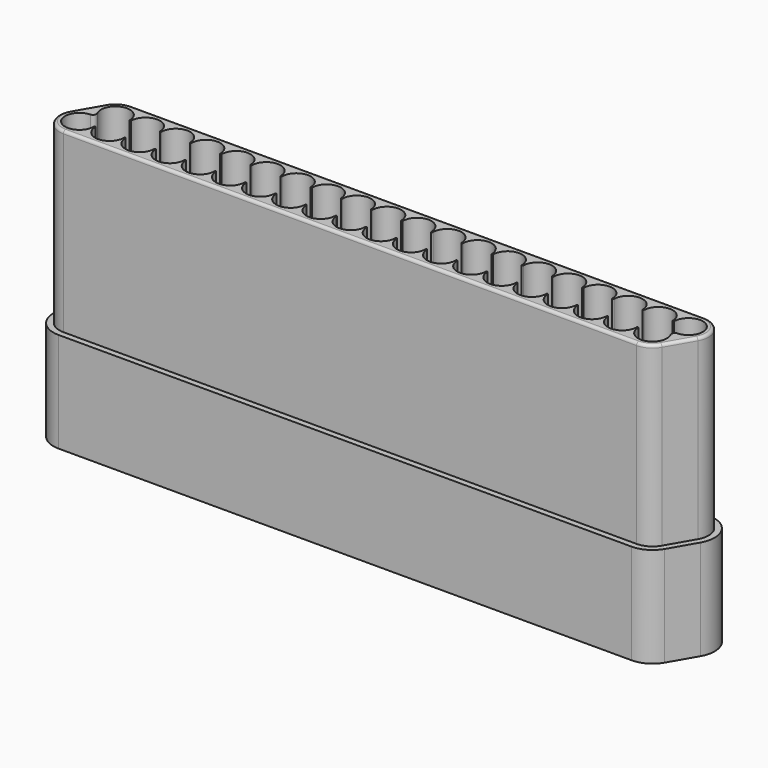
from build123d import *

# Parameters (mm, degrees)
F1_DEPTH = 75
F2_DEPTH = 25
F3_DEPTH = 3.2
F4_R     = 0.8


# Not quite as in the source:
# - a feature names something its author has since deleted; it is built from what else it names


with BuildPart() as f1:
    # F0 (on Top) → F1 (new body)
    with BuildSketch(Plane.XY):
        with BuildLine():
            Line((-0.6430435314, 10.1862159322), (-4.8930435314, 2.825))
            ThreePointArc((-4.8930435314, 2.825), (-4.8930435314, -2.825), (0, -5.65))
            Line((0, -5.65), (161.5, -5.65))
            ThreePointArc((161.5, -5.65), (164.325, -4.8930435314), (166.3930435314, -2.825))
            Line((166.3930435314, -2.825), (170.6430435314, 4.5362159322))
            ThreePointArc((170.6430435314, 4.5362159322), (170.6430435314, 10.1862159322), (165.75, 13.0112159322))
            Line((165.75, 13.0112159322), (4.25, 13.0112159322))
            ThreePointArc((4.25, 13.0112159322), (1.425, 12.2542594635), (-0.6430435314, 10.1862159322))
        make_face()
        with BuildLine():
            ThreePointArc((4.45, 0), (4.25, -0.2), (4.05, 0))
            ThreePointArc((4.05, 0), (-2.7957165477, -2.9302677326), (-0.1902315974, 4.0455298713))
            ThreePointArc((-0.1902315974, 4.0455298713), (0.6288230416, 4.5444261358), (0.651352561, 5.5031963925))
            ThreePointArc((0.651352561, 5.5031963925), (3.2939723142, 11.2967605024), (8.3, 7.3612159322))
            ThreePointArc((8.3, 7.3612159322), (8.5, 7.5612159322), (8.7, 7.3612159322))
            ThreePointArc((8.7, 7.3612159322), (12.75, 11.4112159322), (16.8, 7.3612159322))
            ThreePointArc((16.8, 7.3612159322), (17, 7.5612159322), (17.2, 7.3612159322))
            ThreePointArc((17.2, 7.3612159322), (21.25, 11.4112159322), (25.3, 7.3612159322))
            ThreePointArc((25.3, 7.3612159322), (25.5, 7.5612159322), (25.7, 7.3612159322))
            ThreePointArc((25.7, 7.3612159322), (29.75, 11.4112159322), (33.8, 7.3612159322))
            ThreePointArc((33.8, 7.3612159322), (34, 7.5612159322), (34.2, 7.3612159322))
            ThreePointArc((34.2, 7.3612159322), (38.25, 11.4112159322), (42.3, 7.3612159322))
            ThreePointArc((42.3, 7.3612159322), (42.5, 7.5612159322), (42.7, 7.3612159322))
            ThreePointArc((42.7, 7.3612159322), (46.75, 11.4112159322), (50.8, 7.3612159322))
            ThreePointArc((50.8, 7.3612159322), (51, 7.5612159322), (51.2, 7.3612159322))
            ThreePointArc((51.2, 7.3612159322), (55.25, 11.4112159322), (59.3, 7.3612159322))
            ThreePointArc((59.3, 7.3612159322), (59.5, 7.5612159322), (59.7, 7.3612159322))
            ThreePointArc((59.7, 7.3612159322), (63.75, 11.4112159322), (67.8, 7.3612159322))
            ThreePointArc((67.8, 7.3612159322), (68, 7.5612159322), (68.2, 7.3612159322))
            ThreePointArc((68.2, 7.3612159322), (72.25, 11.4112159322), (76.3, 7.3612159322))
            ThreePointArc((76.3, 7.3612159322), (76.5, 7.5612159322), (76.7, 7.3612159322))
            ThreePointArc((76.7, 7.3612159322), (80.75, 11.4112159322), (84.8, 7.3612159322))
            ThreePointArc((84.8, 7.3612159322), (85, 7.5612159322), (85.2, 7.3612159322))
            ThreePointArc((85.2, 7.3612159322), (89.25, 11.4112159322), (93.3, 7.3612159322))
            ThreePointArc((93.3, 7.3612159322), (93.5, 7.5612159322), (93.7, 7.3612159322))
            ThreePointArc((93.7, 7.3612159322), (97.75, 11.4112159322), (101.8, 7.3612159322))
            ThreePointArc((101.8, 7.3612159322), (102, 7.5612159322), (102.2, 7.3612159322))
            ThreePointArc((102.2, 7.3612159322), (106.25, 11.4112159322), (110.3, 7.3612159322))
            ThreePointArc((110.3, 7.3612159322), (110.5, 7.5612159322), (110.7, 7.3612159322))
            ThreePointArc((110.7, 7.3612159322), (114.75, 11.4112159322), (118.8, 7.3612159322))
            ThreePointArc((118.8, 7.3612159322), (119, 7.5612159322), (119.2, 7.3612159322))
            ThreePointArc((119.2, 7.3612159322), (123.25, 11.4112159322), (127.3, 7.3612159322))
            ThreePointArc((127.3, 7.3612159322), (127.5, 7.5612159322), (127.7, 7.3612159322))
            ThreePointArc((127.7, 7.3612159322), (131.75, 11.4112159322), (135.8, 7.3612159322))
            ThreePointArc((135.8, 7.3612159322), (136, 7.5612159322), (136.2, 7.3612159322))
            ThreePointArc((136.2, 7.3612159322), (140.25, 11.4112159322), (144.3, 7.3612159322))
            ThreePointArc((144.3, 7.3612159322), (144.5, 7.5612159322), (144.7, 7.3612159322))
            ThreePointArc((144.7, 7.3612159322), (148.75, 11.4112159322), (152.8, 7.3612159322))
            ThreePointArc((152.8, 7.3612159322), (153, 7.5612159322), (153.2, 7.3612159322))
            ThreePointArc((153.2, 7.3612159322), (157.25, 11.4112159322), (161.3, 7.3612159322))
            ThreePointArc((161.3, 7.3612159322), (161.5, 7.5612159322), (161.7, 7.3612159322))
            ThreePointArc((161.7, 7.3612159322), (165.75, 11.4112159322), (169.8, 7.3612159322))
            ThreePointArc((169.8, 7.3612159322), (168.6802677326, 4.5654993844), (165.9402315974, 3.3156860609))
            ThreePointArc((165.9402315974, 3.3156860609), (165.1211769584, 2.8167897964), (165.098647439, 1.8580195397))
            ThreePointArc((165.098647439, 1.8580195397), (165.4355445702, 0.9560276858), (165.55, 0))
            ThreePointArc((165.55, 0), (161.5, -4.05), (157.45, 0))
            ThreePointArc((157.45, 0), (157.25, -0.2), (157.05, 0))
            ThreePointArc((157.05, 0), (153, -4.05), (148.95, 0))
            ThreePointArc((148.95, 0), (148.75, -0.2), (148.55, 0))
            ThreePointArc((148.55, 0), (144.5, -4.05), (140.45, 0))
            ThreePointArc((140.45, 0), (140.25, -0.2), (140.05, 0))
            ThreePointArc((140.05, 0), (136, -4.05), (131.95, 0))
            ThreePointArc((131.95, 0), (131.75, -0.2), (131.55, 0))
            ThreePointArc((131.55, 0), (127.5, -4.05), (123.45, 0))
            ThreePointArc((123.45, 0), (123.25, -0.2), (123.05, 0))
            ThreePointArc((123.05, 0), (119, -4.05), (114.95, 0))
            ThreePointArc((114.95, 0), (114.75, -0.2), (114.55, 0))
            ThreePointArc((114.55, 0), (110.5, -4.05), (106.45, 0))
            ThreePointArc((106.45, 0), (106.25, -0.2), (106.05, 0))
            ThreePointArc((106.05, 0), (102, -4.05), (97.95, 0))
            ThreePointArc((97.95, 0), (97.75, -0.2), (97.55, 0))
            ThreePointArc((97.55, 0), (93.5, -4.05), (89.45, 0))
            ThreePointArc((89.45, 0), (89.25, -0.2), (89.05, 0))
            ThreePointArc((89.05, 0), (85, -4.05), (80.95, 0))
            ThreePointArc((80.95, 0), (80.75, -0.2), (80.55, 0))
            ThreePointArc((80.55, 0), (76.5, -4.05), (72.45, 0))
            ThreePointArc((72.45, 0), (72.25, -0.2), (72.05, 0))
            ThreePointArc((72.05, 0), (68, -4.05), (63.95, 0))
            ThreePointArc((63.95, 0), (63.75, -0.2), (63.55, 0))
            ThreePointArc((63.55, 0), (59.5, -4.05), (55.45, 0))
            ThreePointArc((55.45, 0), (55.25, -0.2), (55.05, 0))
            ThreePointArc((55.05, 0), (51, -4.05), (46.95, 0))
            ThreePointArc((46.95, 0), (46.75, -0.2), (46.55, 0))
            ThreePointArc((46.55, 0), (42.5, -4.05), (38.45, 0))
            ThreePointArc((38.45, 0), (38.25, -0.2), (38.05, 0))
            ThreePointArc((38.05, 0), (34, -4.05), (29.95, 0))
            ThreePointArc((29.95, 0), (29.75, -0.2), (29.55, 0))
            ThreePointArc((29.55, 0), (25.5, -4.05), (21.45, 0))
            ThreePointArc((21.45, 0), (21.25, -0.2), (21.05, 0))
            ThreePointArc((21.05, 0), (17, -4.05), (12.95, 0))
            ThreePointArc((12.95, 0), (12.75, -0.2), (12.55, 0))
            ThreePointArc((12.55, 0), (8.5, -4.05), (4.45, 0))
        make_face(mode=Mode.SUBTRACT)
        with BuildLine():
            ThreePointArc((4.45, 0), (4.25, 0.2), (4.05, 0))
            ThreePointArc((4.05, 0), (4.25, -0.2), (4.45, 0))
        make_face()
        with BuildLine():
            ThreePointArc((8.7, 7.3612159322), (8.5, 7.5612159322), (8.3, 7.3612159322))
            ThreePointArc((8.3, 7.3612159322), (8.5, 7.1612159322), (8.7, 7.3612159322))
        make_face()
        with BuildLine():
            ThreePointArc((12.95, 0), (12.75, 0.2), (12.55, 0))
            ThreePointArc((12.55, 0), (12.75, -0.2), (12.95, 0))
        make_face()
        with BuildLine():
            ThreePointArc((17.2, 7.3612159322), (17, 7.5612159322), (16.8, 7.3612159322))
            ThreePointArc((16.8, 7.3612159322), (17, 7.1612159322), (17.2, 7.3612159322))
        make_face()
        with BuildLine():
            ThreePointArc((21.45, 0), (21.25, 0.2), (21.05, 0))
            ThreePointArc((21.05, 0), (21.25, -0.2), (21.45, 0))
        make_face()
        with BuildLine():
            ThreePointArc((25.7, 7.3612159322), (25.5, 7.5612159322), (25.3, 7.3612159322))
            ThreePointArc((25.3, 7.3612159322), (25.5, 7.1612159322), (25.7, 7.3612159322))
        make_face()
        with BuildLine():
            ThreePointArc((29.95, 0), (29.75, 0.2), (29.55, 0))
            ThreePointArc((29.55, 0), (29.75, -0.2), (29.95, 0))
        make_face()
        with BuildLine():
            ThreePointArc((34.2, 7.3612159322), (34, 7.5612159322), (33.8, 7.3612159322))
            ThreePointArc((33.8, 7.3612159322), (34, 7.1612159322), (34.2, 7.3612159322))
        make_face()
        with BuildLine():
            ThreePointArc((38.45, 0), (38.25, 0.2), (38.05, 0))
            ThreePointArc((38.05, 0), (38.25, -0.2), (38.45, 0))
        make_face()
        with BuildLine():
            ThreePointArc((42.7, 7.3612159322), (42.5, 7.5612159322), (42.3, 7.3612159322))
            ThreePointArc((42.3, 7.3612159322), (42.5, 7.1612159322), (42.7, 7.3612159322))
        make_face()
        with BuildLine():
            ThreePointArc((46.95, 0), (46.75, 0.2), (46.55, 0))
            ThreePointArc((46.55, 0), (46.75, -0.2), (46.95, 0))
        make_face()
        with BuildLine():
            ThreePointArc((51.2, 7.3612159322), (51, 7.5612159322), (50.8, 7.3612159322))
            ThreePointArc((50.8, 7.3612159322), (51, 7.1612159322), (51.2, 7.3612159322))
        make_face()
        with BuildLine():
            ThreePointArc((55.45, 0), (55.25, 0.2), (55.05, 0))
            ThreePointArc((55.05, 0), (55.25, -0.2), (55.45, 0))
        make_face()
        with BuildLine():
            ThreePointArc((59.7, 7.3612159322), (59.5, 7.5612159322), (59.3, 7.3612159322))
            ThreePointArc((59.3, 7.3612159322), (59.5, 7.1612159322), (59.7, 7.3612159322))
        make_face()
        with BuildLine():
            ThreePointArc((63.95, 0), (63.75, 0.2), (63.55, 0))
            ThreePointArc((63.55, 0), (63.75, -0.2), (63.95, 0))
        make_face()
        with BuildLine():
            ThreePointArc((68.2, 7.3612159322), (68, 7.5612159322), (67.8, 7.3612159322))
            ThreePointArc((67.8, 7.3612159322), (68, 7.1612159322), (68.2, 7.3612159322))
        make_face()
        with BuildLine():
            ThreePointArc((72.45, 0), (72.25, 0.2), (72.05, 0))
            ThreePointArc((72.05, 0), (72.25, -0.2), (72.45, 0))
        make_face()
        with BuildLine():
            ThreePointArc((76.7, 7.3612159322), (76.5, 7.5612159322), (76.3, 7.3612159322))
            ThreePointArc((76.3, 7.3612159322), (76.5, 7.1612159322), (76.7, 7.3612159322))
        make_face()
        with BuildLine():
            ThreePointArc((80.95, 0), (80.75, 0.2), (80.55, 0))
            ThreePointArc((80.55, 0), (80.75, -0.2), (80.95, 0))
        make_face()
        with BuildLine():
            ThreePointArc((85.2, 7.3612159322), (85, 7.5612159322), (84.8, 7.3612159322))
            ThreePointArc((84.8, 7.3612159322), (85, 7.1612159322), (85.2, 7.3612159322))
        make_face()
        with BuildLine():
            ThreePointArc((89.45, 0), (89.25, 0.2), (89.05, 0))
            ThreePointArc((89.05, 0), (89.25, -0.2), (89.45, 0))
        make_face()
        with BuildLine():
            ThreePointArc((93.7, 7.3612159322), (93.5, 7.5612159322), (93.3, 7.3612159322))
            ThreePointArc((93.3, 7.3612159322), (93.5, 7.1612159322), (93.7, 7.3612159322))
        make_face()
        with BuildLine():
            ThreePointArc((97.95, 0), (97.75, 0.2), (97.55, 0))
            ThreePointArc((97.55, 0), (97.75, -0.2), (97.95, 0))
        make_face()
        with BuildLine():
            ThreePointArc((102.2, 7.3612159322), (102, 7.5612159322), (101.8, 7.3612159322))
            ThreePointArc((101.8, 7.3612159322), (102, 7.1612159322), (102.2, 7.3612159322))
        make_face()
        with BuildLine():
            ThreePointArc((106.45, 0), (106.25, 0.2), (106.05, 0))
            ThreePointArc((106.05, 0), (106.25, -0.2), (106.45, 0))
        make_face()
        with BuildLine():
            ThreePointArc((110.7, 7.3612159322), (110.5, 7.5612159322), (110.3, 7.3612159322))
            ThreePointArc((110.3, 7.3612159322), (110.5, 7.1612159322), (110.7, 7.3612159322))
        make_face()
        with BuildLine():
            ThreePointArc((114.95, 0), (114.75, 0.2), (114.55, 0))
            ThreePointArc((114.55, 0), (114.75, -0.2), (114.95, 0))
        make_face()
        with BuildLine():
            ThreePointArc((119.2, 7.3612159322), (119, 7.5612159322), (118.8, 7.3612159322))
            ThreePointArc((118.8, 7.3612159322), (119, 7.1612159322), (119.2, 7.3612159322))
        make_face()
        with BuildLine():
            ThreePointArc((123.45, 0), (123.25, 0.2), (123.05, 0))
            ThreePointArc((123.05, 0), (123.25, -0.2), (123.45, 0))
        make_face()
        with BuildLine():
            ThreePointArc((127.7, 7.3612159322), (127.5, 7.5612159322), (127.3, 7.3612159322))
            ThreePointArc((127.3, 7.3612159322), (127.5, 7.1612159322), (127.7, 7.3612159322))
        make_face()
        with BuildLine():
            ThreePointArc((131.95, 0), (131.75, 0.2), (131.55, 0))
            ThreePointArc((131.55, 0), (131.75, -0.2), (131.95, 0))
        make_face()
        with BuildLine():
            ThreePointArc((136.2, 7.3612159322), (136, 7.5612159322), (135.8, 7.3612159322))
            ThreePointArc((135.8, 7.3612159322), (136, 7.1612159322), (136.2, 7.3612159322))
        make_face()
        with BuildLine():
            ThreePointArc((140.45, 0), (140.25, 0.2), (140.05, 0))
            ThreePointArc((140.05, 0), (140.25, -0.2), (140.45, 0))
        make_face()
        with BuildLine():
            ThreePointArc((144.7, 7.3612159322), (144.5, 7.5612159322), (144.3, 7.3612159322))
            ThreePointArc((144.3, 7.3612159322), (144.5, 7.1612159322), (144.7, 7.3612159322))
        make_face()
        with BuildLine():
            ThreePointArc((148.95, 0), (148.75, 0.2), (148.55, 0))
            ThreePointArc((148.55, 0), (148.75, -0.2), (148.95, 0))
        make_face()
        with BuildLine():
            ThreePointArc((153.2, 7.3612159322), (153, 7.5612159322), (152.8, 7.3612159322))
            ThreePointArc((152.8, 7.3612159322), (153, 7.1612159322), (153.2, 7.3612159322))
        make_face()
        with BuildLine():
            ThreePointArc((157.45, 0), (157.25, 0.2), (157.05, 0))
            ThreePointArc((157.05, 0), (157.25, -0.2), (157.45, 0))
        make_face()
        with BuildLine():
            ThreePointArc((161.7, 7.3612159322), (161.5, 7.5612159322), (161.3, 7.3612159322))
            ThreePointArc((161.3, 7.3612159322), (161.5, 7.1612159322), (161.7, 7.3612159322))
        make_face()
    extrude(amount=F1_DEPTH)

    # F0 (on Top) → F2 (join)
    with BuildSketch(Plane.XY):
        with BuildLine():
            Line((-2.1152867178, 11.0362159322), (-6.3652867178, 3.675))
            ThreePointArc((-6.3652867178, 3.675), (-6.3652867178, -3.675), (0, -7.35))
            Line((0, -7.35), (161.5, -7.35))
            ThreePointArc((161.5, -7.35), (165.175, -6.3652867178), (167.8652867178, -3.675))
            Line((167.8652867178, -3.675), (172.1152867178, 3.6862159322))
            ThreePointArc((172.1152867178, 3.6862159322), (172.1152867178, 11.0362159322), (165.75, 14.7112159322))
            Line((165.75, 14.7112159322), (4.25, 14.7112159322))
            ThreePointArc((4.25, 14.7112159322), (0.575, 13.72650265), (-2.1152867178, 11.0362159322))
        make_face()
        with BuildLine():
            ThreePointArc((0, -5.65), (-4.8930435314, -2.825), (-4.8930435314, 2.825))
            Line((-4.8930435314, 2.825), (-0.6430435314, 10.1862159322))
            ThreePointArc((-0.6430435314, 10.1862159322), (1.425, 12.2542594635), (4.25, 13.0112159322))
            Line((4.25, 13.0112159322), (165.75, 13.0112159322))
            ThreePointArc((165.75, 13.0112159322), (170.6430435314, 10.1862159322), (170.6430435314, 4.5362159322))
            Line((170.6430435314, 4.5362159322), (166.3930435314, -2.825))
            ThreePointArc((166.3930435314, -2.825), (164.325, -4.8930435314), (161.5, -5.65))
            Line((161.5, -5.65), (0, -5.65))
        make_face(mode=Mode.SUBTRACT)
    extrude(amount=F2_DEPTH)

    # F0 (on Top) → F3 (join)
    with BuildSketch(Plane.XY):
        with BuildLine():
            Line((-2.1152867178, 11.0362159322), (-6.3652867178, 3.675))
            ThreePointArc((-6.3652867178, 3.675), (-6.3652867178, -3.675), (0, -7.35))
            Line((0, -7.35), (161.5, -7.35))
            ThreePointArc((161.5, -7.35), (165.175, -6.3652867178), (167.8652867178, -3.675))
            Line((167.8652867178, -3.675), (172.1152867178, 3.6862159322))
            ThreePointArc((172.1152867178, 3.6862159322), (172.1152867178, 11.0362159322), (165.75, 14.7112159322))
            Line((165.75, 14.7112159322), (4.25, 14.7112159322))
            ThreePointArc((4.25, 14.7112159322), (0.575, 13.72650265), (-2.1152867178, 11.0362159322))
        make_face()
        with BuildLine():
            ThreePointArc((0, -5.65), (-4.8930435314, -2.825), (-4.8930435314, 2.825))
            Line((-4.8930435314, 2.825), (-0.6430435314, 10.1862159322))
            ThreePointArc((-0.6430435314, 10.1862159322), (1.425, 12.2542594635), (4.25, 13.0112159322))
            Line((4.25, 13.0112159322), (165.75, 13.0112159322))
            ThreePointArc((165.75, 13.0112159322), (170.6430435314, 10.1862159322), (170.6430435314, 4.5362159322))
            Line((170.6430435314, 4.5362159322), (166.3930435314, -2.825))
            ThreePointArc((166.3930435314, -2.825), (164.325, -4.8930435314), (161.5, -5.65))
            Line((161.5, -5.65), (0, -5.65))
        make_face(mode=Mode.SUBTRACT)
        with BuildLine():
            Line((-0.6430435314, 10.1862159322), (-4.8930435314, 2.825))
            ThreePointArc((-4.8930435314, 2.825), (-4.8930435314, -2.825), (0, -5.65))
            Line((0, -5.65), (161.5, -5.65))
            ThreePointArc((161.5, -5.65), (164.325, -4.8930435314), (166.3930435314, -2.825))
            Line((166.3930435314, -2.825), (170.6430435314, 4.5362159322))
            ThreePointArc((170.6430435314, 4.5362159322), (170.6430435314, 10.1862159322), (165.75, 13.0112159322))
            Line((165.75, 13.0112159322), (4.25, 13.0112159322))
            ThreePointArc((4.25, 13.0112159322), (1.425, 12.2542594635), (-0.6430435314, 10.1862159322))
        make_face()
        with BuildLine():
            ThreePointArc((4.45, 0), (4.25, -0.2), (4.05, 0))
            ThreePointArc((4.05, 0), (-2.7957165477, -2.9302677326), (-0.1902315974, 4.0455298713))
            ThreePointArc((-0.1902315974, 4.0455298713), (0.6288230416, 4.5444261358), (0.651352561, 5.5031963925))
            ThreePointArc((0.651352561, 5.5031963925), (3.2939723142, 11.2967605024), (8.3, 7.3612159322))
            ThreePointArc((8.3, 7.3612159322), (8.5, 7.5612159322), (8.7, 7.3612159322))
            ThreePointArc((8.7, 7.3612159322), (12.75, 11.4112159322), (16.8, 7.3612159322))
            ThreePointArc((16.8, 7.3612159322), (17, 7.5612159322), (17.2, 7.3612159322))
            ThreePointArc((17.2, 7.3612159322), (21.25, 11.4112159322), (25.3, 7.3612159322))
            ThreePointArc((25.3, 7.3612159322), (25.5, 7.5612159322), (25.7, 7.3612159322))
            ThreePointArc((25.7, 7.3612159322), (29.75, 11.4112159322), (33.8, 7.3612159322))
            ThreePointArc((33.8, 7.3612159322), (34, 7.5612159322), (34.2, 7.3612159322))
            ThreePointArc((34.2, 7.3612159322), (38.25, 11.4112159322), (42.3, 7.3612159322))
            ThreePointArc((42.3, 7.3612159322), (42.5, 7.5612159322), (42.7, 7.3612159322))
            ThreePointArc((42.7, 7.3612159322), (46.75, 11.4112159322), (50.8, 7.3612159322))
            ThreePointArc((50.8, 7.3612159322), (51, 7.5612159322), (51.2, 7.3612159322))
            ThreePointArc((51.2, 7.3612159322), (55.25, 11.4112159322), (59.3, 7.3612159322))
            ThreePointArc((59.3, 7.3612159322), (59.5, 7.5612159322), (59.7, 7.3612159322))
            ThreePointArc((59.7, 7.3612159322), (63.75, 11.4112159322), (67.8, 7.3612159322))
            ThreePointArc((67.8, 7.3612159322), (68, 7.5612159322), (68.2, 7.3612159322))
            ThreePointArc((68.2, 7.3612159322), (72.25, 11.4112159322), (76.3, 7.3612159322))
            ThreePointArc((76.3, 7.3612159322), (76.5, 7.5612159322), (76.7, 7.3612159322))
            ThreePointArc((76.7, 7.3612159322), (80.75, 11.4112159322), (84.8, 7.3612159322))
            ThreePointArc((84.8, 7.3612159322), (85, 7.5612159322), (85.2, 7.3612159322))
            ThreePointArc((85.2, 7.3612159322), (89.25, 11.4112159322), (93.3, 7.3612159322))
            ThreePointArc((93.3, 7.3612159322), (93.5, 7.5612159322), (93.7, 7.3612159322))
            ThreePointArc((93.7, 7.3612159322), (97.75, 11.4112159322), (101.8, 7.3612159322))
            ThreePointArc((101.8, 7.3612159322), (102, 7.5612159322), (102.2, 7.3612159322))
            ThreePointArc((102.2, 7.3612159322), (106.25, 11.4112159322), (110.3, 7.3612159322))
            ThreePointArc((110.3, 7.3612159322), (110.5, 7.5612159322), (110.7, 7.3612159322))
            ThreePointArc((110.7, 7.3612159322), (114.75, 11.4112159322), (118.8, 7.3612159322))
            ThreePointArc((118.8, 7.3612159322), (119, 7.5612159322), (119.2, 7.3612159322))
            ThreePointArc((119.2, 7.3612159322), (123.25, 11.4112159322), (127.3, 7.3612159322))
            ThreePointArc((127.3, 7.3612159322), (127.5, 7.5612159322), (127.7, 7.3612159322))
            ThreePointArc((127.7, 7.3612159322), (131.75, 11.4112159322), (135.8, 7.3612159322))
            ThreePointArc((135.8, 7.3612159322), (136, 7.5612159322), (136.2, 7.3612159322))
            ThreePointArc((136.2, 7.3612159322), (140.25, 11.4112159322), (144.3, 7.3612159322))
            ThreePointArc((144.3, 7.3612159322), (144.5, 7.5612159322), (144.7, 7.3612159322))
            ThreePointArc((144.7, 7.3612159322), (148.75, 11.4112159322), (152.8, 7.3612159322))
            ThreePointArc((152.8, 7.3612159322), (153, 7.5612159322), (153.2, 7.3612159322))
            ThreePointArc((153.2, 7.3612159322), (157.25, 11.4112159322), (161.3, 7.3612159322))
            ThreePointArc((161.3, 7.3612159322), (161.5, 7.5612159322), (161.7, 7.3612159322))
            ThreePointArc((161.7, 7.3612159322), (165.75, 11.4112159322), (169.8, 7.3612159322))
            ThreePointArc((169.8, 7.3612159322), (168.6802677326, 4.5654993844), (165.9402315974, 3.3156860609))
            ThreePointArc((165.9402315974, 3.3156860609), (165.1211769584, 2.8167897964), (165.098647439, 1.8580195397))
            ThreePointArc((165.098647439, 1.8580195397), (165.4355445702, 0.9560276858), (165.55, 0))
            ThreePointArc((165.55, 0), (161.5, -4.05), (157.45, 0))
            ThreePointArc((157.45, 0), (157.25, -0.2), (157.05, 0))
            ThreePointArc((157.05, 0), (153, -4.05), (148.95, 0))
            ThreePointArc((148.95, 0), (148.75, -0.2), (148.55, 0))
            ThreePointArc((148.55, 0), (144.5, -4.05), (140.45, 0))
            ThreePointArc((140.45, 0), (140.25, -0.2), (140.05, 0))
            ThreePointArc((140.05, 0), (136, -4.05), (131.95, 0))
            ThreePointArc((131.95, 0), (131.75, -0.2), (131.55, 0))
            ThreePointArc((131.55, 0), (127.5, -4.05), (123.45, 0))
            ThreePointArc((123.45, 0), (123.25, -0.2), (123.05, 0))
            ThreePointArc((123.05, 0), (119, -4.05), (114.95, 0))
            ThreePointArc((114.95, 0), (114.75, -0.2), (114.55, 0))
            ThreePointArc((114.55, 0), (110.5, -4.05), (106.45, 0))
            ThreePointArc((106.45, 0), (106.25, -0.2), (106.05, 0))
            ThreePointArc((106.05, 0), (102, -4.05), (97.95, 0))
            ThreePointArc((97.95, 0), (97.75, -0.2), (97.55, 0))
            ThreePointArc((97.55, 0), (93.5, -4.05), (89.45, 0))
            ThreePointArc((89.45, 0), (89.25, -0.2), (89.05, 0))
            ThreePointArc((89.05, 0), (85, -4.05), (80.95, 0))
            ThreePointArc((80.95, 0), (80.75, -0.2), (80.55, 0))
            ThreePointArc((80.55, 0), (76.5, -4.05), (72.45, 0))
            ThreePointArc((72.45, 0), (72.25, -0.2), (72.05, 0))
            ThreePointArc((72.05, 0), (68, -4.05), (63.95, 0))
            ThreePointArc((63.95, 0), (63.75, -0.2), (63.55, 0))
            ThreePointArc((63.55, 0), (59.5, -4.05), (55.45, 0))
            ThreePointArc((55.45, 0), (55.25, -0.2), (55.05, 0))
            ThreePointArc((55.05, 0), (51, -4.05), (46.95, 0))
            ThreePointArc((46.95, 0), (46.75, -0.2), (46.55, 0))
            ThreePointArc((46.55, 0), (42.5, -4.05), (38.45, 0))
            ThreePointArc((38.45, 0), (38.25, -0.2), (38.05, 0))
            ThreePointArc((38.05, 0), (34, -4.05), (29.95, 0))
            ThreePointArc((29.95, 0), (29.75, -0.2), (29.55, 0))
            ThreePointArc((29.55, 0), (25.5, -4.05), (21.45, 0))
            ThreePointArc((21.45, 0), (21.25, -0.2), (21.05, 0))
            ThreePointArc((21.05, 0), (17, -4.05), (12.95, 0))
            ThreePointArc((12.95, 0), (12.75, -0.2), (12.55, 0))
            ThreePointArc((12.55, 0), (8.5, -4.05), (4.45, 0))
        make_face(mode=Mode.SUBTRACT)
        with BuildLine():
            ThreePointArc((-0.1902315974, 4.0455298713), (2.7957165477, 2.9302677326), (4.05, 0))
            ThreePointArc((4.05, 0), (4.25, 0.2), (4.45, 0))
            ThreePointArc((4.45, 0), (8.5, 4.05), (12.55, 0))
            ThreePointArc((12.55, 0), (12.75, 0.2), (12.95, 0))
            ThreePointArc((12.95, 0), (17, 4.05), (21.05, 0))
            ThreePointArc((21.05, 0), (21.25, 0.2), (21.45, 0))
            ThreePointArc((21.45, 0), (25.5, 4.05), (29.55, 0))
            ThreePointArc((29.55, 0), (29.75, 0.2), (29.95, 0))
            ThreePointArc((29.95, 0), (34, 4.05), (38.05, 0))
            ThreePointArc((38.05, 0), (38.25, 0.2), (38.45, 0))
            ThreePointArc((38.45, 0), (42.5, 4.05), (46.55, 0))
            ThreePointArc((46.55, 0), (46.75, 0.2), (46.95, 0))
            ThreePointArc((46.95, 0), (51, 4.05), (55.05, 0))
            ThreePointArc((55.05, 0), (55.25, 0.2), (55.45, 0))
            ThreePointArc((55.45, 0), (59.5, 4.05), (63.55, 0))
            ThreePointArc((63.55, 0), (63.75, 0.2), (63.95, 0))
            ThreePointArc((63.95, 0), (68, 4.05), (72.05, 0))
            ThreePointArc((72.05, 0), (72.25, 0.2), (72.45, 0))
            ThreePointArc((72.45, 0), (76.5, 4.05), (80.55, 0))
            ThreePointArc((80.55, 0), (80.75, 0.2), (80.95, 0))
            ThreePointArc((80.95, 0), (85, 4.05), (89.05, 0))
            ThreePointArc((89.05, 0), (89.25, 0.2), (89.45, 0))
            ThreePointArc((89.45, 0), (93.5, 4.05), (97.55, 0))
            ThreePointArc((97.55, 0), (97.75, 0.2), (97.95, 0))
            ThreePointArc((97.95, 0), (102, 4.05), (106.05, 0))
            ThreePointArc((106.05, 0), (106.25, 0.2), (106.45, 0))
            ThreePointArc((106.45, 0), (110.5, 4.05), (114.55, 0))
            ThreePointArc((114.55, 0), (114.75, 0.2), (114.95, 0))
            ThreePointArc((114.95, 0), (119, 4.05), (123.05, 0))
            ThreePointArc((123.05, 0), (123.25, 0.2), (123.45, 0))
            ThreePointArc((123.45, 0), (127.5, 4.05), (131.55, 0))
            ThreePointArc((131.55, 0), (131.75, 0.2), (131.95, 0))
            ThreePointArc((131.95, 0), (136, 4.05), (140.05, 0))
            ThreePointArc((140.05, 0), (140.25, 0.2), (140.45, 0))
            ThreePointArc((140.45, 0), (144.5, 4.05), (148.55, 0))
            ThreePointArc((148.55, 0), (148.75, 0.2), (148.95, 0))
            ThreePointArc((148.95, 0), (153, 4.05), (157.05, 0))
            ThreePointArc((157.05, 0), (157.25, 0.2), (157.45, 0))
            ThreePointArc((157.45, 0), (160.5439723142, 3.9355445702), (165.098647439, 1.8580195397))
            ThreePointArc((165.098647439, 1.8580195397), (165.1211769584, 2.8167897964), (165.9402315974, 3.3156860609))
            ThreePointArc((165.9402315974, 3.3156860609), (162.9542834523, 4.4309481996), (161.7, 7.3612159322))
            ThreePointArc((161.7, 7.3612159322), (161.5, 7.1612159322), (161.3, 7.3612159322))
            ThreePointArc((161.3, 7.3612159322), (157.25, 3.3112159322), (153.2, 7.3612159322))
            ThreePointArc((153.2, 7.3612159322), (153, 7.1612159322), (152.8, 7.3612159322))
            ThreePointArc((152.8, 7.3612159322), (148.75, 3.3112159322), (144.7, 7.3612159322))
            ThreePointArc((144.7, 7.3612159322), (144.5, 7.1612159322), (144.3, 7.3612159322))
            ThreePointArc((144.3, 7.3612159322), (140.25, 3.3112159322), (136.2, 7.3612159322))
            ThreePointArc((136.2, 7.3612159322), (136, 7.1612159322), (135.8, 7.3612159322))
            ThreePointArc((135.8, 7.3612159322), (131.75, 3.3112159322), (127.7, 7.3612159322))
            ThreePointArc((127.7, 7.3612159322), (127.5, 7.1612159322), (127.3, 7.3612159322))
            ThreePointArc((127.3, 7.3612159322), (123.25, 3.3112159322), (119.2, 7.3612159322))
            ThreePointArc((119.2, 7.3612159322), (119, 7.1612159322), (118.8, 7.3612159322))
            ThreePointArc((118.8, 7.3612159322), (114.75, 3.3112159322), (110.7, 7.3612159322))
            ThreePointArc((110.7, 7.3612159322), (110.5, 7.1612159322), (110.3, 7.3612159322))
            ThreePointArc((110.3, 7.3612159322), (106.25, 3.3112159322), (102.2, 7.3612159322))
            ThreePointArc((102.2, 7.3612159322), (102, 7.1612159322), (101.8, 7.3612159322))
            ThreePointArc((101.8, 7.3612159322), (97.75, 3.3112159322), (93.7, 7.3612159322))
            ThreePointArc((93.7, 7.3612159322), (93.5, 7.1612159322), (93.3, 7.3612159322))
            ThreePointArc((93.3, 7.3612159322), (89.25, 3.3112159322), (85.2, 7.3612159322))
            ThreePointArc((85.2, 7.3612159322), (85, 7.1612159322), (84.8, 7.3612159322))
            ThreePointArc((84.8, 7.3612159322), (80.75, 3.3112159322), (76.7, 7.3612159322))
            ThreePointArc((76.7, 7.3612159322), (76.5, 7.1612159322), (76.3, 7.3612159322))
            ThreePointArc((76.3, 7.3612159322), (72.25, 3.3112159322), (68.2, 7.3612159322))
            ThreePointArc((68.2, 7.3612159322), (68, 7.1612159322), (67.8, 7.3612159322))
            ThreePointArc((67.8, 7.3612159322), (63.75, 3.3112159322), (59.7, 7.3612159322))
            ThreePointArc((59.7, 7.3612159322), (59.5, 7.1612159322), (59.3, 7.3612159322))
            ThreePointArc((59.3, 7.3612159322), (55.25, 3.3112159322), (51.2, 7.3612159322))
            ThreePointArc((51.2, 7.3612159322), (51, 7.1612159322), (50.8, 7.3612159322))
            ThreePointArc((50.8, 7.3612159322), (46.75, 3.3112159322), (42.7, 7.3612159322))
            ThreePointArc((42.7, 7.3612159322), (42.5, 7.1612159322), (42.3, 7.3612159322))
            ThreePointArc((42.3, 7.3612159322), (38.25, 3.3112159322), (34.2, 7.3612159322))
            ThreePointArc((34.2, 7.3612159322), (34, 7.1612159322), (33.8, 7.3612159322))
            ThreePointArc((33.8, 7.3612159322), (29.75, 3.3112159322), (25.7, 7.3612159322))
            ThreePointArc((25.7, 7.3612159322), (25.5, 7.1612159322), (25.3, 7.3612159322))
            ThreePointArc((25.3, 7.3612159322), (21.25, 3.3112159322), (17.2, 7.3612159322))
            ThreePointArc((17.2, 7.3612159322), (17, 7.1612159322), (16.8, 7.3612159322))
            ThreePointArc((16.8, 7.3612159322), (12.75, 3.3112159322), (8.7, 7.3612159322))
            ThreePointArc((8.7, 7.3612159322), (8.5, 7.1612159322), (8.3, 7.3612159322))
            ThreePointArc((8.3, 7.3612159322), (5.2060276858, 3.425671362), (0.651352561, 5.5031963925))
            ThreePointArc((0.651352561, 5.5031963925), (0.6288230416, 4.5444261358), (-0.1902315974, 4.0455298713))
        make_face()
        with BuildLine():
            ThreePointArc((-0.1902315974, 4.0455298713), (-2.7957165477, -2.9302677326), (4.05, 0))
            ThreePointArc((4.05, 0), (2.7957165477, 2.9302677326), (-0.1902315974, 4.0455298713))
        make_face()
        with BuildLine():
            ThreePointArc((12.55, 0), (8.5, 4.05), (4.45, 0))
            ThreePointArc((4.45, 0), (8.5, -4.05), (12.55, 0))
        make_face()
        with BuildLine():
            ThreePointArc((8.3, 7.3612159322), (3.2939723142, 11.2967605024), (0.651352561, 5.5031963925))
            ThreePointArc((0.651352561, 5.5031963925), (5.2060276858, 3.425671362), (8.3, 7.3612159322))
        make_face()
        with BuildLine():
            ThreePointArc((21.05, 0), (17, 4.05), (12.95, 0))
            ThreePointArc((12.95, 0), (17, -4.05), (21.05, 0))
        make_face()
        with BuildLine():
            ThreePointArc((16.8, 7.3612159322), (12.75, 11.4112159322), (8.7, 7.3612159322))
            ThreePointArc((8.7, 7.3612159322), (12.75, 3.3112159322), (16.8, 7.3612159322))
        make_face()
        with BuildLine():
            ThreePointArc((29.55, 0), (25.5, 4.05), (21.45, 0))
            ThreePointArc((21.45, 0), (25.5, -4.05), (29.55, 0))
        make_face()
        with BuildLine():
            ThreePointArc((25.3, 7.3612159322), (21.25, 11.4112159322), (17.2, 7.3612159322))
            ThreePointArc((17.2, 7.3612159322), (21.25, 3.3112159322), (25.3, 7.3612159322))
        make_face()
        with BuildLine():
            ThreePointArc((38.05, 0), (34, 4.05), (29.95, 0))
            ThreePointArc((29.95, 0), (34, -4.05), (38.05, 0))
        make_face()
        with BuildLine():
            ThreePointArc((33.8, 7.3612159322), (29.75, 11.4112159322), (25.7, 7.3612159322))
            ThreePointArc((25.7, 7.3612159322), (29.75, 3.3112159322), (33.8, 7.3612159322))
        make_face()
        with BuildLine():
            ThreePointArc((46.55, 0), (42.5, 4.05), (38.45, 0))
            ThreePointArc((38.45, 0), (42.5, -4.05), (46.55, 0))
        make_face()
        with BuildLine():
            ThreePointArc((42.3, 7.3612159322), (38.25, 11.4112159322), (34.2, 7.3612159322))
            ThreePointArc((34.2, 7.3612159322), (38.25, 3.3112159322), (42.3, 7.3612159322))
        make_face()
        with BuildLine():
            ThreePointArc((55.05, 0), (51, 4.05), (46.95, 0))
            ThreePointArc((46.95, 0), (51, -4.05), (55.05, 0))
        make_face()
        with BuildLine():
            ThreePointArc((50.8, 7.3612159322), (46.75, 11.4112159322), (42.7, 7.3612159322))
            ThreePointArc((42.7, 7.3612159322), (46.75, 3.3112159322), (50.8, 7.3612159322))
        make_face()
        with BuildLine():
            ThreePointArc((63.55, 0), (59.5, 4.05), (55.45, 0))
            ThreePointArc((55.45, 0), (59.5, -4.05), (63.55, 0))
        make_face()
        with BuildLine():
            ThreePointArc((59.3, 7.3612159322), (55.25, 11.4112159322), (51.2, 7.3612159322))
            ThreePointArc((51.2, 7.3612159322), (55.25, 3.3112159322), (59.3, 7.3612159322))
        make_face()
        with BuildLine():
            ThreePointArc((72.05, 0), (68, 4.05), (63.95, 0))
            ThreePointArc((63.95, 0), (68, -4.05), (72.05, 0))
        make_face()
        with BuildLine():
            ThreePointArc((67.8, 7.3612159322), (63.75, 11.4112159322), (59.7, 7.3612159322))
            ThreePointArc((59.7, 7.3612159322), (63.75, 3.3112159322), (67.8, 7.3612159322))
        make_face()
        with BuildLine():
            ThreePointArc((80.55, 0), (76.5, 4.05), (72.45, 0))
            ThreePointArc((72.45, 0), (76.5, -4.05), (80.55, 0))
        make_face()
        with BuildLine():
            ThreePointArc((76.3, 7.3612159322), (72.25, 11.4112159322), (68.2, 7.3612159322))
            ThreePointArc((68.2, 7.3612159322), (72.25, 3.3112159322), (76.3, 7.3612159322))
        make_face()
        with BuildLine():
            ThreePointArc((89.05, 0), (85, 4.05), (80.95, 0))
            ThreePointArc((80.95, 0), (85, -4.05), (89.05, 0))
        make_face()
        with BuildLine():
            ThreePointArc((84.8, 7.3612159322), (80.75, 11.4112159322), (76.7, 7.3612159322))
            ThreePointArc((76.7, 7.3612159322), (80.75, 3.3112159322), (84.8, 7.3612159322))
        make_face()
        with BuildLine():
            ThreePointArc((97.55, 0), (93.5, 4.05), (89.45, 0))
            ThreePointArc((89.45, 0), (93.5, -4.05), (97.55, 0))
        make_face()
        with BuildLine():
            ThreePointArc((93.3, 7.3612159322), (89.25, 11.4112159322), (85.2, 7.3612159322))
            ThreePointArc((85.2, 7.3612159322), (89.25, 3.3112159322), (93.3, 7.3612159322))
        make_face()
        with BuildLine():
            ThreePointArc((106.05, 0), (102, 4.05), (97.95, 0))
            ThreePointArc((97.95, 0), (102, -4.05), (106.05, 0))
        make_face()
        with BuildLine():
            ThreePointArc((101.8, 7.3612159322), (97.75, 11.4112159322), (93.7, 7.3612159322))
            ThreePointArc((93.7, 7.3612159322), (97.75, 3.3112159322), (101.8, 7.3612159322))
        make_face()
        with BuildLine():
            ThreePointArc((114.55, 0), (110.5, 4.05), (106.45, 0))
            ThreePointArc((106.45, 0), (110.5, -4.05), (114.55, 0))
        make_face()
        with BuildLine():
            ThreePointArc((110.3, 7.3612159322), (106.25, 11.4112159322), (102.2, 7.3612159322))
            ThreePointArc((102.2, 7.3612159322), (106.25, 3.3112159322), (110.3, 7.3612159322))
        make_face()
        with BuildLine():
            ThreePointArc((123.05, 0), (119, 4.05), (114.95, 0))
            ThreePointArc((114.95, 0), (119, -4.05), (123.05, 0))
        make_face()
        with BuildLine():
            ThreePointArc((118.8, 7.3612159322), (114.75, 11.4112159322), (110.7, 7.3612159322))
            ThreePointArc((110.7, 7.3612159322), (114.75, 3.3112159322), (118.8, 7.3612159322))
        make_face()
        with BuildLine():
            ThreePointArc((131.55, 0), (127.5, 4.05), (123.45, 0))
            ThreePointArc((123.45, 0), (127.5, -4.05), (131.55, 0))
        make_face()
        with BuildLine():
            ThreePointArc((127.3, 7.3612159322), (123.25, 11.4112159322), (119.2, 7.3612159322))
            ThreePointArc((119.2, 7.3612159322), (123.25, 3.3112159322), (127.3, 7.3612159322))
        make_face()
        with BuildLine():
            ThreePointArc((140.05, 0), (136, 4.05), (131.95, 0))
            ThreePointArc((131.95, 0), (136, -4.05), (140.05, 0))
        make_face()
        with BuildLine():
            ThreePointArc((135.8, 7.3612159322), (131.75, 11.4112159322), (127.7, 7.3612159322))
            ThreePointArc((127.7, 7.3612159322), (131.75, 3.3112159322), (135.8, 7.3612159322))
        make_face()
        with BuildLine():
            ThreePointArc((148.55, 0), (144.5, 4.05), (140.45, 0))
            ThreePointArc((140.45, 0), (144.5, -4.05), (148.55, 0))
        make_face()
        with BuildLine():
            ThreePointArc((144.3, 7.3612159322), (140.25, 11.4112159322), (136.2, 7.3612159322))
            ThreePointArc((136.2, 7.3612159322), (140.25, 3.3112159322), (144.3, 7.3612159322))
        make_face()
        with BuildLine():
            ThreePointArc((157.05, 0), (153, 4.05), (148.95, 0))
            ThreePointArc((148.95, 0), (153, -4.05), (157.05, 0))
        make_face()
        with BuildLine():
            ThreePointArc((152.8, 7.3612159322), (148.75, 11.4112159322), (144.7, 7.3612159322))
            ThreePointArc((144.7, 7.3612159322), (148.75, 3.3112159322), (152.8, 7.3612159322))
        make_face()
        with BuildLine():
            ThreePointArc((165.098647439, 1.8580195397), (160.5439723142, 3.9355445702), (157.45, 0))
            ThreePointArc((157.45, 0), (161.5, -4.05), (165.55, 0))
            ThreePointArc((165.55, 0), (165.4355445702, 0.9560276858), (165.098647439, 1.8580195397))
        make_face()
        with BuildLine():
            ThreePointArc((161.3, 7.3612159322), (157.25, 11.4112159322), (153.2, 7.3612159322))
            ThreePointArc((153.2, 7.3612159322), (157.25, 3.3112159322), (161.3, 7.3612159322))
        make_face()
        with BuildLine():
            ThreePointArc((161.7, 7.3612159322), (162.9542834523, 4.4309481996), (165.9402315974, 3.3156860609))
            ThreePointArc((165.9402315974, 3.3156860609), (168.6802677326, 4.5654993844), (169.8, 7.3612159322))
            ThreePointArc((169.8, 7.3612159322), (165.75, 11.4112159322), (161.7, 7.3612159322))
        make_face()
        with BuildLine():
            ThreePointArc((4.45, 0), (4.25, 0.2), (4.05, 0))
            ThreePointArc((4.05, 0), (4.25, -0.2), (4.45, 0))
        make_face()
        with BuildLine():
            ThreePointArc((12.95, 0), (12.75, 0.2), (12.55, 0))
            ThreePointArc((12.55, 0), (12.75, -0.2), (12.95, 0))
        make_face()
        with BuildLine():
            ThreePointArc((8.7, 7.3612159322), (8.5, 7.5612159322), (8.3, 7.3612159322))
            ThreePointArc((8.3, 7.3612159322), (8.5, 7.1612159322), (8.7, 7.3612159322))
        make_face()
        with BuildLine():
            ThreePointArc((21.45, 0), (21.25, 0.2), (21.05, 0))
            ThreePointArc((21.05, 0), (21.25, -0.2), (21.45, 0))
        make_face()
        with BuildLine():
            ThreePointArc((17.2, 7.3612159322), (17, 7.5612159322), (16.8, 7.3612159322))
            ThreePointArc((16.8, 7.3612159322), (17, 7.1612159322), (17.2, 7.3612159322))
        make_face()
        with BuildLine():
            ThreePointArc((29.95, 0), (29.75, 0.2), (29.55, 0))
            ThreePointArc((29.55, 0), (29.75, -0.2), (29.95, 0))
        make_face()
        with BuildLine():
            ThreePointArc((25.7, 7.3612159322), (25.5, 7.5612159322), (25.3, 7.3612159322))
            ThreePointArc((25.3, 7.3612159322), (25.5, 7.1612159322), (25.7, 7.3612159322))
        make_face()
        with BuildLine():
            ThreePointArc((38.45, 0), (38.25, 0.2), (38.05, 0))
            ThreePointArc((38.05, 0), (38.25, -0.2), (38.45, 0))
        make_face()
        with BuildLine():
            ThreePointArc((34.2, 7.3612159322), (34, 7.5612159322), (33.8, 7.3612159322))
            ThreePointArc((33.8, 7.3612159322), (34, 7.1612159322), (34.2, 7.3612159322))
        make_face()
        with BuildLine():
            ThreePointArc((46.95, 0), (46.75, 0.2), (46.55, 0))
            ThreePointArc((46.55, 0), (46.75, -0.2), (46.95, 0))
        make_face()
        with BuildLine():
            ThreePointArc((42.7, 7.3612159322), (42.5, 7.5612159322), (42.3, 7.3612159322))
            ThreePointArc((42.3, 7.3612159322), (42.5, 7.1612159322), (42.7, 7.3612159322))
        make_face()
        with BuildLine():
            ThreePointArc((55.45, 0), (55.25, 0.2), (55.05, 0))
            ThreePointArc((55.05, 0), (55.25, -0.2), (55.45, 0))
        make_face()
        with BuildLine():
            ThreePointArc((51.2, 7.3612159322), (51, 7.5612159322), (50.8, 7.3612159322))
            ThreePointArc((50.8, 7.3612159322), (51, 7.1612159322), (51.2, 7.3612159322))
        make_face()
        with BuildLine():
            ThreePointArc((63.95, 0), (63.75, 0.2), (63.55, 0))
            ThreePointArc((63.55, 0), (63.75, -0.2), (63.95, 0))
        make_face()
        with BuildLine():
            ThreePointArc((59.7, 7.3612159322), (59.5, 7.5612159322), (59.3, 7.3612159322))
            ThreePointArc((59.3, 7.3612159322), (59.5, 7.1612159322), (59.7, 7.3612159322))
        make_face()
        with BuildLine():
            ThreePointArc((72.45, 0), (72.25, 0.2), (72.05, 0))
            ThreePointArc((72.05, 0), (72.25, -0.2), (72.45, 0))
        make_face()
        with BuildLine():
            ThreePointArc((68.2, 7.3612159322), (68, 7.5612159322), (67.8, 7.3612159322))
            ThreePointArc((67.8, 7.3612159322), (68, 7.1612159322), (68.2, 7.3612159322))
        make_face()
        with BuildLine():
            ThreePointArc((80.95, 0), (80.75, 0.2), (80.55, 0))
            ThreePointArc((80.55, 0), (80.75, -0.2), (80.95, 0))
        make_face()
        with BuildLine():
            ThreePointArc((76.7, 7.3612159322), (76.5, 7.5612159322), (76.3, 7.3612159322))
            ThreePointArc((76.3, 7.3612159322), (76.5, 7.1612159322), (76.7, 7.3612159322))
        make_face()
        with BuildLine():
            ThreePointArc((89.45, 0), (89.25, 0.2), (89.05, 0))
            ThreePointArc((89.05, 0), (89.25, -0.2), (89.45, 0))
        make_face()
        with BuildLine():
            ThreePointArc((85.2, 7.3612159322), (85, 7.5612159322), (84.8, 7.3612159322))
            ThreePointArc((84.8, 7.3612159322), (85, 7.1612159322), (85.2, 7.3612159322))
        make_face()
        with BuildLine():
            ThreePointArc((97.95, 0), (97.75, 0.2), (97.55, 0))
            ThreePointArc((97.55, 0), (97.75, -0.2), (97.95, 0))
        make_face()
        with BuildLine():
            ThreePointArc((93.7, 7.3612159322), (93.5, 7.5612159322), (93.3, 7.3612159322))
            ThreePointArc((93.3, 7.3612159322), (93.5, 7.1612159322), (93.7, 7.3612159322))
        make_face()
        with BuildLine():
            ThreePointArc((106.45, 0), (106.25, 0.2), (106.05, 0))
            ThreePointArc((106.05, 0), (106.25, -0.2), (106.45, 0))
        make_face()
        with BuildLine():
            ThreePointArc((102.2, 7.3612159322), (102, 7.5612159322), (101.8, 7.3612159322))
            ThreePointArc((101.8, 7.3612159322), (102, 7.1612159322), (102.2, 7.3612159322))
        make_face()
        with BuildLine():
            ThreePointArc((114.95, 0), (114.75, 0.2), (114.55, 0))
            ThreePointArc((114.55, 0), (114.75, -0.2), (114.95, 0))
        make_face()
        with BuildLine():
            ThreePointArc((110.7, 7.3612159322), (110.5, 7.5612159322), (110.3, 7.3612159322))
            ThreePointArc((110.3, 7.3612159322), (110.5, 7.1612159322), (110.7, 7.3612159322))
        make_face()
        with BuildLine():
            ThreePointArc((123.45, 0), (123.25, 0.2), (123.05, 0))
            ThreePointArc((123.05, 0), (123.25, -0.2), (123.45, 0))
        make_face()
        with BuildLine():
            ThreePointArc((119.2, 7.3612159322), (119, 7.5612159322), (118.8, 7.3612159322))
            ThreePointArc((118.8, 7.3612159322), (119, 7.1612159322), (119.2, 7.3612159322))
        make_face()
        with BuildLine():
            ThreePointArc((131.95, 0), (131.75, 0.2), (131.55, 0))
            ThreePointArc((131.55, 0), (131.75, -0.2), (131.95, 0))
        make_face()
        with BuildLine():
            ThreePointArc((127.7, 7.3612159322), (127.5, 7.5612159322), (127.3, 7.3612159322))
            ThreePointArc((127.3, 7.3612159322), (127.5, 7.1612159322), (127.7, 7.3612159322))
        make_face()
        with BuildLine():
            ThreePointArc((140.45, 0), (140.25, 0.2), (140.05, 0))
            ThreePointArc((140.05, 0), (140.25, -0.2), (140.45, 0))
        make_face()
        with BuildLine():
            ThreePointArc((136.2, 7.3612159322), (136, 7.5612159322), (135.8, 7.3612159322))
            ThreePointArc((135.8, 7.3612159322), (136, 7.1612159322), (136.2, 7.3612159322))
        make_face()
        with BuildLine():
            ThreePointArc((148.95, 0), (148.75, 0.2), (148.55, 0))
            ThreePointArc((148.55, 0), (148.75, -0.2), (148.95, 0))
        make_face()
        with BuildLine():
            ThreePointArc((144.7, 7.3612159322), (144.5, 7.5612159322), (144.3, 7.3612159322))
            ThreePointArc((144.3, 7.3612159322), (144.5, 7.1612159322), (144.7, 7.3612159322))
        make_face()
        with BuildLine():
            ThreePointArc((157.45, 0), (157.25, 0.2), (157.05, 0))
            ThreePointArc((157.05, 0), (157.25, -0.2), (157.45, 0))
        make_face()
        with BuildLine():
            ThreePointArc((153.2, 7.3612159322), (153, 7.5612159322), (152.8, 7.3612159322))
            ThreePointArc((152.8, 7.3612159322), (153, 7.1612159322), (153.2, 7.3612159322))
        make_face()
        with BuildLine():
            ThreePointArc((161.7, 7.3612159322), (161.5, 7.5612159322), (161.3, 7.3612159322))
            ThreePointArc((161.3, 7.3612159322), (161.5, 7.1612159322), (161.7, 7.3612159322))
        make_face()
    extrude(amount=-F3_DEPTH)

    # F4
    f4_edges = [f1.edges().sort_by_distance(p)[0] for p in [
        (80.75, -5.65, 75),
        (170.643044, 10.186216, 75),
        (168.518044, 0.855608, 75),
        (164.325, -4.893044, 75),
        (-4.893044, -2.825, 75),
        (-2.768044, 6.505608, 75),
        (1.425, 12.254259, 75),
        (85, 13.011216, 75),
    ]]
    fillet(f4_edges, radius=F4_R)


solid = f1.part
